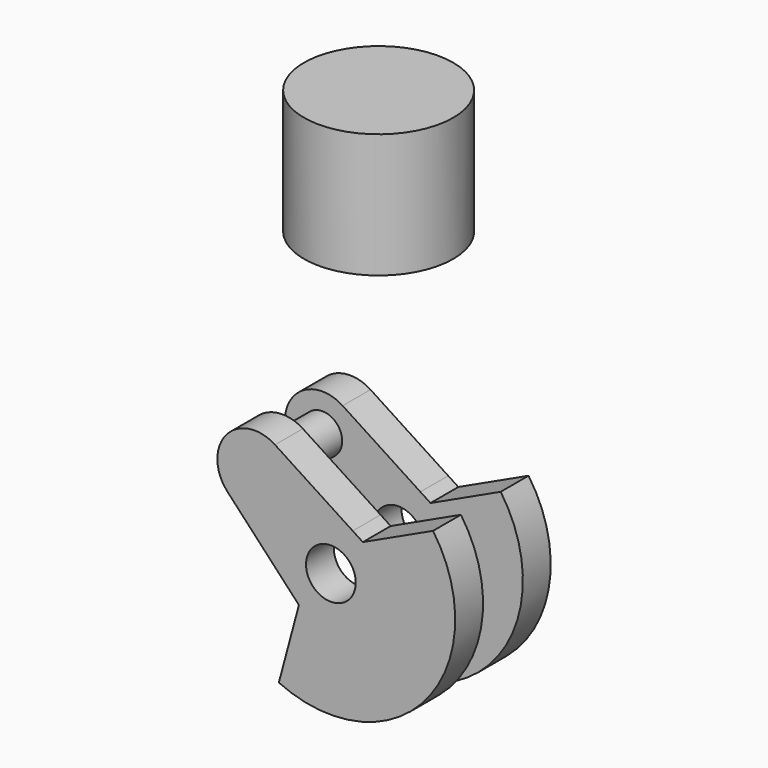
from build123d import *

# Parameters (mm, degrees)
F2_W          = 15
F2_H          = 25
F4_T          = -3
F0_W          = 10
F0_H          = 7
F5_DEPTH      = 13.0000001
F5_DEPTH_BACK = 13.0000001
F1_R          = 5
F1_R_2        = 4
F6_DEPTH      = 12
F6_DEPTH_BACK = 12
F7_DEPTH      = 12
F8_DEPTH      = 5
F9_DEPTH      = 5


with BuildPart() as f3:
    # F2 (on Front) → F3 (revolve)
    with BuildSketch(Plane.XZ):
        with Locations((7.5, 68.178761995)):
            Rectangle(F2_W, F2_H)
    revolve(axis=Axis((0, 0, -11.7868287861), (0, 0, -1)))

    # F4
    f4_openings = [f3.faces().sort_by_distance(p)[0] for p in [
        (0, 0, 55.678762),
    ]]
    offset(amount=F4_T, openings=f4_openings)

    # F0 (on Front) → F5 (join, two sides)
    with BuildSketch(Plane.XZ) as f5_sk:
        with Locations((0, 77.178761995)):
            Rectangle(F0_W, F0_H)
        with BuildLine():
            Line((5, 73.678761995), (-5, 73.678761995))
            Line((-5, 73.678761995), (-5, 65.678761995))
            ThreePointArc((-5, 65.678761995), (-3.9977518928, 62.6757668562), (-1.3928080784, 60.8766701949))
            ThreePointArc((-1.3928080784, 60.8766701949), (3.0029951389, 61.6810101023), (5, 65.678761995))
            Line((5, 65.678761995), (5, 73.678761995))
        make_face()
        with BuildLine():
            ThreePointArc((2.5, 65.678761995), (1.5014975694, 63.6798860486), (-0.6964040392, 63.277716095))
            ThreePointArc((-0.6964040392, 63.277716095), (-1.5014975694, 67.6776379414), (2.5, 65.678761995))
        make_face(mode=Mode.SUBTRACT)
    extrude(amount=F5_DEPTH)
    extrude(f5_sk.sketch, amount=-F5_DEPTH_BACK)

    # F0 (on Front) → F8 (cut, symmetric)
    with BuildSketch(Plane.XZ):
        with BuildLine():
            Line((5, 73.678761995), (-5, 73.678761995))
            Line((-5, 73.678761995), (-5, 65.678761995))
            ThreePointArc((-5, 65.678761995), (-3.9977518928, 62.6757668562), (-1.3928080784, 60.8766701949))
            ThreePointArc((-1.3928080784, 60.8766701949), (3.0029951389, 61.6810101023), (5, 65.678761995))
            Line((5, 65.678761995), (5, 73.678761995))
        make_face()
        with BuildLine():
            ThreePointArc((2.5, 65.678761995), (1.5014975694, 63.6798860486), (-0.6964040392, 63.277716095))
            ThreePointArc((-0.6964040392, 63.277716095), (-1.5014975694, 67.6776379414), (2.5, 65.678761995))
        make_face(mode=Mode.SUBTRACT)
    extrude(amount=F8_DEPTH, both=True, mode=Mode.SUBTRACT)


with BuildPart() as f6:
    # F1 (on Front) → F6 (new body, two sides)
    with BuildSketch(Plane.XZ) as f6_sk:
        with BuildLine():
            Line((20.545541793, 14.2436200606), (6.4278760969, 7.6604444312))
            ThreePointArc((6.4278760969, 7.6604444312), (9.0630778704, 4.2261826174), (10, 0))
            ThreePointArc((10, 0), (4.2261826174, -9.0630778704), (-6.4278760969, -7.6604444312))
            Line((-6.4278760969, -7.6604444312), (-10.4595315751, -22.7067875145))
            ThreePointArc((-10.4595315751, -22.7067875145), (19.151111078, -16.0696902422), (20.545541793, 14.2436200606))
        make_face()
        with BuildLine():
            Line((6.4278760969, 7.6604444312), (4.3938839854, 8.9829718647))
            ThreePointArc((4.3938839854, 8.9829718647), (-7.6604444312, 6.4278760969), (-8.0835103905, -5.887007709))
            Line((-8.0835103905, -5.887007709), (-6.4278760969, -7.6604444312))
            ThreePointArc((-6.4278760969, -7.6604444312), (4.2261826174, -9.0630778704), (10, 0))
            ThreePointArc((10, 0), (9.0630778704, 4.2261826174), (6.4278760969, 7.6604444312))
        make_face()
        Circle(F1_R, mode=Mode.SUBTRACT)
        with BuildLine():
            ThreePointArc((-11.2325362548, 19.1434682303), (-8.7287479144, 16.4325772833), (-7.8208888624, 12.8557521937))
            ThreePointArc((-7.8208888624, 12.8557521937), (-12.5701547705, 5.8783986872), (-20.8031453839, 7.7376604173))
            Line((-20.8031453839, 7.7376604173), (-8.0835103905, -5.887007709))
            ThreePointArc((-8.0835103905, -5.887007709), (-7.6604444312, 6.4278760969), (4.3938839854, 8.9829718647))
            Line((4.3938839854, 8.9829718647), (-11.2325362548, 19.1434682303))
        make_face()
        with BuildLine():
            ThreePointArc((-20.8031453839, 7.7376604173), (-12.5701547705, 5.8783986872), (-7.8208888624, 12.8557521937))
            ThreePointArc((-7.8208888624, 12.8557521937), (-8.7287479144, 16.4325772833), (-11.2325362548, 19.1434682303))
            ThreePointArc((-11.2325362548, 19.1434682303), (-21.0662221858, 17.6766592664), (-20.8031453839, 7.7376604173))
        make_face()
        with Locations((-15.3208888624, 12.8557521937)):
            Circle(F1_R_2, mode=Mode.SUBTRACT)
    extrude(amount=F6_DEPTH)
    extrude(f6_sk.sketch, amount=-F6_DEPTH_BACK)

    # F1 (on Front) → F7 (join, symmetric)
    with BuildSketch(Plane.XZ):
        with Locations((-15.3208888624, 12.8557521937)):
            Circle(F1_R_2)
    extrude(amount=F7_DEPTH, both=True)

    # F1 (on Front) → F9 (cut, symmetric)
    with BuildSketch(Plane.XZ):
        with BuildLine():
            Line((20.545541793, 14.2436200606), (6.4278760969, 7.6604444312))
            ThreePointArc((6.4278760969, 7.6604444312), (9.0630778704, 4.2261826174), (10, 0))
            ThreePointArc((10, 0), (4.2261826174, -9.0630778704), (-6.4278760969, -7.6604444312))
            Line((-6.4278760969, -7.6604444312), (-10.4595315751, -22.7067875145))
            ThreePointArc((-10.4595315751, -22.7067875145), (19.151111078, -16.0696902422), (20.545541793, 14.2436200606))
        make_face()
        with BuildLine():
            ThreePointArc((-11.2325362548, 19.1434682303), (-8.7287479144, 16.4325772833), (-7.8208888624, 12.8557521937))
            ThreePointArc((-7.8208888624, 12.8557521937), (-12.5701547705, 5.8783986872), (-20.8031453839, 7.7376604173))
            Line((-20.8031453839, 7.7376604173), (-8.0835103905, -5.887007709))
            ThreePointArc((-8.0835103905, -5.887007709), (-7.6604444312, 6.4278760969), (4.3938839854, 8.9829718647))
            Line((4.3938839854, 8.9829718647), (-11.2325362548, 19.1434682303))
        make_face()
        with BuildLine():
            ThreePointArc((-20.8031453839, 7.7376604173), (-12.5701547705, 5.8783986872), (-7.8208888624, 12.8557521937))
            ThreePointArc((-7.8208888624, 12.8557521937), (-8.7287479144, 16.4325772833), (-11.2325362548, 19.1434682303))
            ThreePointArc((-11.2325362548, 19.1434682303), (-21.0662221858, 17.6766592664), (-20.8031453839, 7.7376604173))
        make_face()
        with Locations((-15.3208888624, 12.8557521937)):
            Circle(F1_R_2, mode=Mode.SUBTRACT)
        with BuildLine():
            Line((6.4278760969, 7.6604444312), (4.3938839854, 8.9829718647))
            ThreePointArc((4.3938839854, 8.9829718647), (-7.6604444312, 6.4278760969), (-8.0835103905, -5.887007709))
            Line((-8.0835103905, -5.887007709), (-6.4278760969, -7.6604444312))
            ThreePointArc((-6.4278760969, -7.6604444312), (4.2261826174, -9.0630778704), (10, 0))
            ThreePointArc((10, 0), (9.0630778704, 4.2261826174), (6.4278760969, 7.6604444312))
        make_face()
        Circle(F1_R, mode=Mode.SUBTRACT)
    extrude(amount=F9_DEPTH, both=True, mode=Mode.SUBTRACT)


solid = Compound([f3.part, f6.part])
